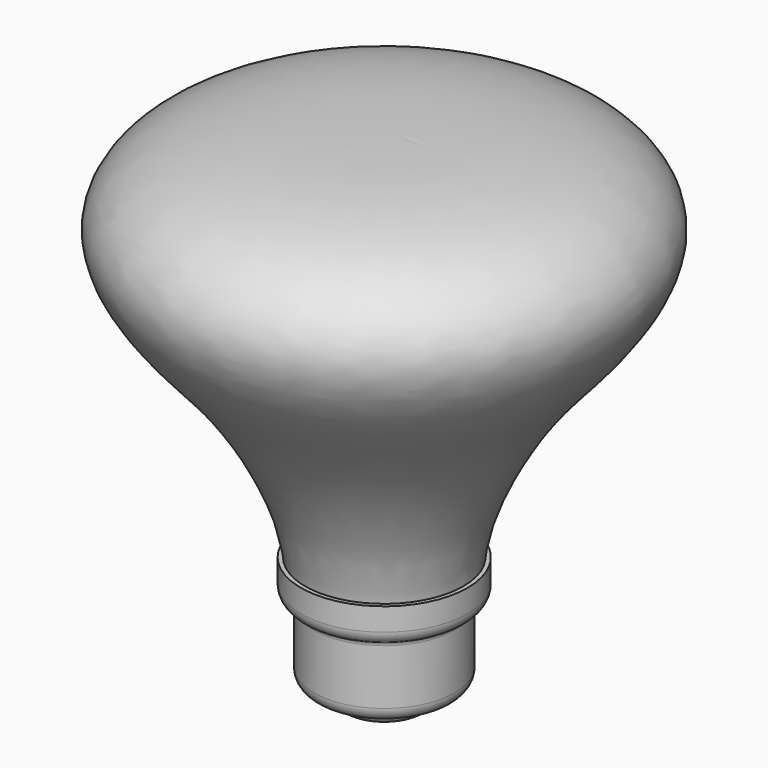
from build123d import *


# Not quite as in the source:
# - ends of sketch curves that miss each other by under 0.0002 mm in the source are joined
# - the dataset's text gives a spline's control points without its knots; the knots are read off the source's solid


with BuildPart() as f1:
    # F0 (on Front) → F1 (revolve)
    with BuildSketch(Plane.XZ):
        with BuildLine():
            add(Edge.make_bspline(
                [(0, 95), (11.9351603372, 95), (35.8246105824, 94.6516896617), (48.8877822791, 78.5166303587), (36.7335882746, 61.259762649), (25.6252541946, 50.5859582932), (15.715134495, 31.5667555555), (15.0648372379, 23.3361808845)],
                knots=[0, 0, 0, 0, 0.2515012998, 0.4180438437, 0.5951767558, 0.7721555554, 0.985957916, 0.985957916, 0.985957916, 0.985957916], degree=3))
            Line((0, 95), (0, 94))
            add(Edge.make_bspline(
                [(0, 94), (2.9630700502, 94), (9.1782743728, 93.9740433972), (18.6538919368, 93.5132289158), (26.0693555428, 92.4954189536), (31.3398035501, 91.1418374515), (34.8630183202, 89.8252494458), (37.8754907722, 88.1720131282), (40.3436552409, 86.230602179), (42.2181089779, 84.0653509783), (43.4655047768, 81.7360020156), (43.9642983461, 79.6929781768), (44.0236023298, 78.0105778888), (43.8523999941, 76.2739630041), (43.2373588823, 74.0093258938), (41.9684089943, 71.2232368208), (40.3051479186, 68.4504963203), (38.3928330992, 65.7659370649), (36.3769457009, 63.2357259813), (34.4109131489, 60.9305910363), (32.4718958327, 58.7349470211), (30.5295002512, 56.5240708444), (28.5601548126, 54.1790088041), (26.8783194447, 52.0145084957), (25.4984431135, 50.0997277455), (24.4420222221, 48.554820116), (23.371206791, 46.9041625925), (21.9423543159, 44.5821782467), (20.184673887, 41.4832470787), (18.2217979455, 37.5529247559), (16.5063594028, 33.5123322099), (14.7441069739, 28.2806941544), (14.059053557, 24.5166496304), (14.0054439278, 22.2091477859)],
                knots=[0, 0, 0, 0, 0.0625, 0.125, 0.1875, 0.21875, 0.25, 0.28125, 0.3125, 0.34375, 0.375, 0.40625, 0.421875, 0.4375, 0.46875, 0.5, 0.53125, 0.5625, 0.59375, 0.625, 0.65625, 0.6875, 0.71875, 0.75, 0.765625, 0.78125, 0.796875, 0.8125, 0.84375, 0.875, 0.90625, 0.9375, 0.9960505799, 0.9960505799, 0.9960505799, 0.9960505799], degree=3))
            Line((14.0054439278, 22.2091477859), (11.4234326196, 19.9979832119))
            Line((11.4234326196, 19.9979832119), (12.1221662313, 19.2797821416))
            Line((12.1221662313, 19.2797821416), (13.6790529308, 20.6130328355))
            ThreePointArc((13.6790529308, 20.6130328355), (14.6422054295, 21.8370739244), (15.0648372379, 23.3361808845))
        make_face()
    revolve(axis=Axis((0, 0, 47.5), (0, 0, 1)))


with BuildPart() as f3:
    # F2 (on Front) → F3 (revolve)
    with BuildSketch(Plane.XZ):
        with BuildLine():
            Line((15.8648372379, 23.3361808845), (15.0648372379, 23.3361808845))
            Line((15.0648372379, 23.3361808845), (15.0648372379, 18.9961523027))
            ThreePointArc((15.0648372379, 18.9961523027), (14.8164462053, 18.0308202224), (14.1329712125, 17.3052679743))
            Line((14.1329712125, 17.3052679743), (13.560167464, 16.9434270522))
            ThreePointArc((13.560167464, 16.9434270522), (12.8766924712, 16.2178748041), (12.6283014386, 15.2525427237))
            Line((12.6283014386, 15.2525427237), (12.6283014386, 4.947202207))
            ThreePointArc((12.6283014386, 4.947202207), (12.1987252529, 3.7087479109), (11.094532395, 3.0023040875))
            Line((11.094532395, 3.0023040875), (8.0580403753, 2.274396253))
            ThreePointArc((8.0580403753, 2.274396253), (7.5059439464, 1.9211743413), (7.2911558535, 1.3019471932))
            Line((7.2911558535, 1.3019471932), (7.2911558535, 1))
            ThreePointArc((7.2911558535, 1), (6.9982626347, 0.2928932188), (6.2911558535, 0))
            Line((6.2911558535, 0), (0, 0))
            Line((0, 0), (0, -0.8))
            Line((0, -0.8), (6.2911558535, -0.8))
            ThreePointArc((6.2911558535, -0.8), (7.7129791776, -0.1038199288), (8.0349746538, 1.4462017387))
            Line((8.0349746538, 1.4462017387), (11.2810247776, 2.2243448397))
            ThreePointArc((11.2810247776, 2.2243448397), (12.8268947786, 3.2133661924), (13.4283014386, 4.947202207))
            Line((13.4283014386, 4.947202207), (13.4283014386, 15.4491866455))
            ThreePointArc((13.4283014386, 15.4491866455), (13.6040422656, 16.0153993403), (14.06949507, 16.3825986606))
            ThreePointArc((14.06949507, 16.3825986606), (15.3727629224, 17.4107567574), (15.8648372379, 18.9961523027))
            Line((15.8648372379, 18.9961523027), (15.8648372379, 23.3361808845))
        make_face()
    revolve(axis=Axis((0, 0, 11.6680904422), (0, 0, 1)))


solid = Compound([f1.part, f3.part])
